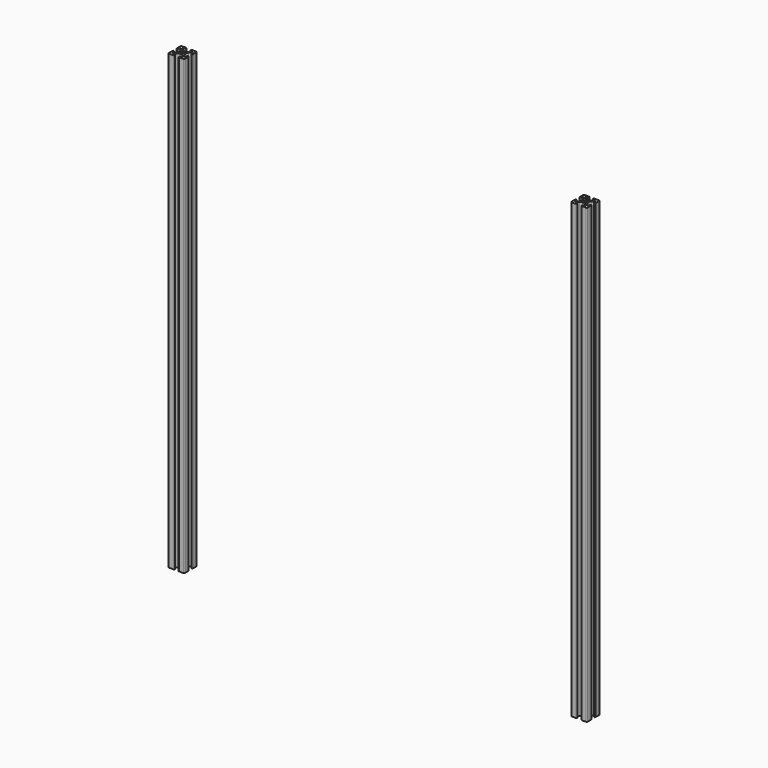
from build123d import *

# Parameters (mm, degrees)
F0_R     = 2.6035
F1_DEPTH = 713.74
F2_R     = 1.18109
F3_R     = 5.08
F4_R     = 0.762
F5_R     = 1.27


# Not quite as in the source:
# - a fillet or chamfer is up to 0.001 mm smaller than in the source, because OpenCascade refuses the exact size


with BuildPart() as f1:
    # F0 (on Top) → F1 (new body)
    with BuildSketch(Plane.XY):
        Polygon((12.7, 3.2385), (12.7, 12.7), (3.2385, 12.7), (3.2385, 10.3378), (8.7752354349, 10.3378), (2.9459354349, 4.5085), (-2.9459354349, 4.5085), (-8.7752354349, 10.3378), (-3.2385, 10.3378), (-3.2385, 12.7), (-12.7, 12.7), (-12.7, 3.2385), (-10.3378, 3.2385), (-10.3378, 8.7752354349), (-4.5085, 2.9459354349), (-4.5085, -2.9459354349), (-10.3378, -8.7752354349), (-10.3378, -3.2385), (-12.7, -3.2385), (-12.7, -12.7), (-3.2385, -12.7), (-3.2385, -10.3378), (-8.7752354349, -10.3378), (-2.9459354349, -4.5085), (2.9459354349, -4.5085), (8.7752354349, -10.3378), (3.2385, -10.3378), (3.2385, -12.7), (12.7, -12.7), (12.7, -3.2385), (10.3378, -3.2385), (10.3378, -8.7752354349), (4.5085, -2.9459354349), (4.5085, 2.9459354349), (10.3378, 8.7752354349), (10.3378, 3.2385), align=None)
        Circle(F0_R, mode=Mode.SUBTRACT)
    extrude(amount=F1_DEPTH)

    # F2 (radius 1.1811 in the source; OpenCascade refuses exactly that, so slightly less here)
    f2_edges = [f1.edges().sort_by_distance(p)[0] for p in [
        (3.2385, 12.7, 356.87),
        (3.2385, 10.3378, 356.87),
        (-3.2385, 12.7, 356.87),
        (-12.7, 3.2385, 356.87),
        (-3.2385, 10.3378, 356.87),
        (-10.3378, 3.2385, 356.87),
        (12.7, 3.2385, 356.87),
        (10.3378, 3.2385, 356.87),
        (12.7, -3.2385, 356.87),
        (10.3378, -3.2385, 356.87),
        (3.2385, -10.3378, 356.87),
        (-3.2385, -10.3378, 356.87),
        (-10.3378, -3.2385, 356.87),
        (-12.7, -3.2385, 356.87),
        (-3.2385, -12.7, 356.87),
        (3.2385, -12.7, 356.87),
    ]]
    fillet(f2_edges, radius=F2_R)

    # F3
    f3_edges = [f1.edges().sort_by_distance(p)[0] for p in [
        (2.945935, 4.5085, 356.87),
        (-2.945935, 4.5085, 356.87),
        (4.5085, -2.945935, 356.87),
        (4.5085, 2.945935, 356.87),
        (2.945935, -4.5085, 356.87),
        (-2.945935, -4.5085, 356.87),
        (-4.5085, -2.945935, 356.87),
        (-4.5085, 2.945935, 356.87),
    ]]
    fillet(f3_edges, radius=F3_R)

    # F4
    f4_edges = [f1.edges().sort_by_distance(p)[0] for p in [
        (8.775235, 10.3378, 356.87),
        (-8.775235, 10.3378, 356.87),
        (-10.3378, 8.775235, 356.87),
        (-10.3378, -8.775235, 356.87),
        (-8.775235, -10.3378, 356.87),
        (8.775235, -10.3378, 356.87),
        (10.3378, -8.775235, 356.87),
        (10.3378, 8.775235, 356.87),
    ]]
    fillet(f4_edges, radius=F4_R)

    # F5
    f5_edges = [f1.edges().sort_by_distance(p)[0] for p in [
        (-12.7, -12.7, 356.87),
        (12.7, -12.7, 356.87),
        (12.7, 12.7, 356.87),
        (-12.7, 12.7, 356.87),
    ]]
    fillet(f5_edges, radius=F5_R)


with BuildPart() as f6_1:
    # F6: copy of F1
    add(f1.part.moved(Location((635, 0, 0))))


solid = Compound([f1.part, f6_1.part])
